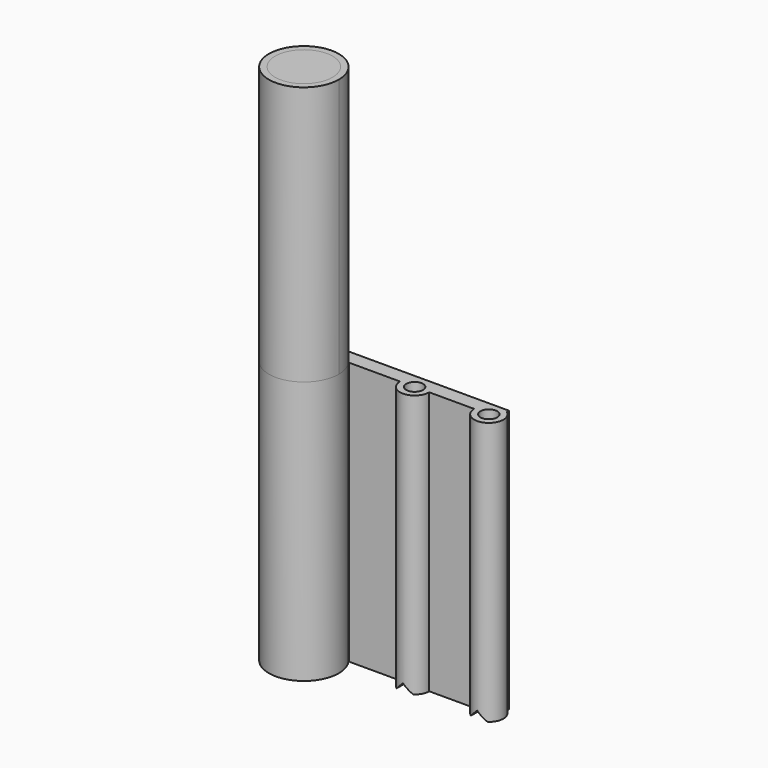
from build123d import *
from build123d import SkipClean  # not in build123d's __all__

# Parameters (mm, degrees)
F0_R     = 6
F0_R_2   = 1.75
F1_DEPTH = 109.2
F3_DEPTH = 25
F4_W     = 51.9569627941
F4_H     = 21.8115057796
F4_R     = 7.3
F5_DEPTH = 54.2
F6_R     = 6
F7_DEPTH = 1.2


with BuildPart() as f1:
    # F0 (on Top) → F1 (new body)
    with BuildSketch(Plane.XY):
        with BuildLine():
            Line((-1.3, -1.8418754227), (-1.3, -1.75))
            Line((-1.3, -1.75), (9.4, -1.75))
            ThreePointArc((9.4, -1.75), (12.45, -4.8), (15.5, -1.75))
            Line((15.5, -1.75), (24.9, -1.75))
            ThreePointArc((24.9, -1.75), (29.358012784, -4.4555498517), (29.7, 0.7479991994))
            Line((29.7, 0.7479991994), (29.7, 1.3))
            Line((29.7, 1.3), (-13.3, 1.3))
            Line((-13.3, 1.3), (-13.3, -1.8418754227))
            ThreePointArc((-13.3, -1.8418754227), (-7.3, -13.3), (-1.3, -1.8418754227))
        make_face()
        with Locations((-7.3, -6)):
            Circle(F0_R, mode=Mode.SUBTRACT)
        with Locations((12.45, -1.75)):
            Circle(F0_R_2, mode=Mode.SUBTRACT)
        with Locations((27.95, -1.75)):
            Circle(F0_R_2, mode=Mode.SUBTRACT)
    extrude(amount=F1_DEPTH)

    # F2 (on face) → F3 (cut)
    with BuildSketch(Plane.XZ.offset(1.75)):
        Polygon((12.45, 1.75), (10.7, 0), (14.2, 0), align=None)
        Polygon((27.95, 1.75), (26.2, 0), (29.7, 0), align=None)
    extrude(amount=F3_DEPTH, mode=Mode.SUBTRACT)

    # F4 (on face) → F5 (cut)
    with BuildSketch(Plane.XY.offset(109.2)):
        with Locations((7.5893197209, -5.5296784267)):
            Rectangle(F4_W, F4_H)
        with Locations((-7.3, -6)):
            Circle(F4_R, mode=Mode.SUBTRACT)
    with SkipClean():  # cleaning this boolean's faces spoils the solid; the shape is the same uncleaned
        extrude(amount=-F5_DEPTH, mode=Mode.SUBTRACT)


with BuildPart() as f7:
    # F6 (on face) → F7 (new body)
    with BuildSketch(Plane.XY.offset(109.2)):
        with Locations((-7.3, -6)):
            Circle(F6_R)
    extrude(amount=-F7_DEPTH)


solid = Compound([f1.part, f7.part])
